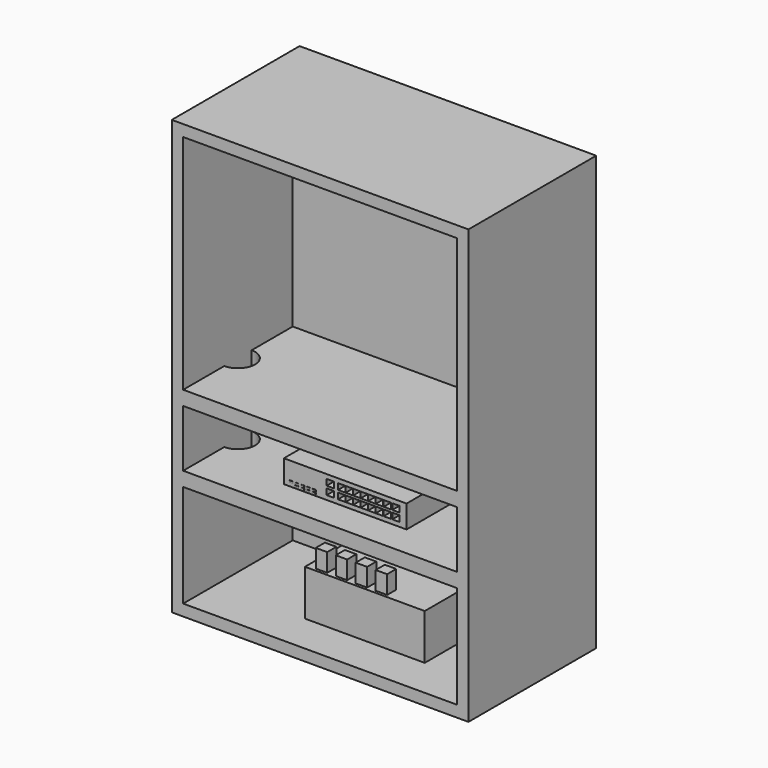
from build123d import *

# Parameters (mm, degrees)
F0_W      = 660.4
F0_H      = 355.6
F1_DEPTH  = 965.2
F2_W      = 609.6
F2_H      = 914.4
F3_DEPTH  = 304.8
F4_W      = 609.6
F4_H      = 31.75
F5_DEPTH  = 304.8
F6_W      = 266.7
F6_H      = 152.4
F7_DEPTH  = 101.6
F8_W      = 25.4
F8_H      = 25.4
F9_DEPTH  = 40.64
F10_W     = 273.05
F10_H     = 215.9
F11_DEPTH = 50.8
F12_W     = 16
F12_H     = 13.3
F13_DEPTH = 19.05
F12_W_2   = 7.62
F12_H_2   = 3.81
F14_DEPTH = 0.635
F16_DEPTH = 190.5


# Not quite as in the source:
# - a feature names something its author has since deleted; it is built from what else it names


with BuildPart() as f1:
    # F0 (on Top) → F1 (new body)
    with BuildSketch(Plane.XY):
        Rectangle(F0_W, F0_H)
    extrude(amount=F1_DEPTH)

    # F2 (on face) → F3 (cut)
    with BuildSketch(Plane.XZ.offset(177.8)):
        with Locations((0, 482.6)):
            Rectangle(F2_W, F2_H)
    extrude(amount=-F3_DEPTH, mode=Mode.SUBTRACT)

    # F4 (on face) → F5 (join)
    with BuildSketch(Plane.XZ.offset(-127)):
        with Locations((0, 269.875)):
            Rectangle(F4_W, F4_H)
        with Locations((0, 428.625)):
            Rectangle(F4_W, F4_H)
    extrude(amount=F5_DEPTH)

    # F6 (on face) → F7 (join)
    with BuildSketch(Plane.XY.offset(25.4)):
        with Locations((29.1608499646, -13.5529870272)):
            Rectangle(F6_W, F6_H)
    extrude(amount=F7_DEPTH)

    # F8 (on face) → F9 (join)
    with BuildSketch(Plane.XY.offset(127)):
        with Locations((-72.4391500354, -70.7029870272)):
            Rectangle(F8_W, F8_H)
        with Locations((-72.4391500354, 43.5970129728)):
            Rectangle(F8_W, F8_H)
        with Locations((-27.9891500354, -70.7029870272)):
            Rectangle(F8_W, F8_H)
        with Locations((-27.9891500354, 43.5970129728)):
            Rectangle(F8_W, F8_H)
        with Locations((16.4608499646, -70.7029870272)):
            Rectangle(F8_W, F8_H)
        with Locations((16.4608499646, 43.5970129728)):
            Rectangle(F8_W, F8_H)
        with Locations((60.9108499646, -70.7029870272)):
            Rectangle(F8_W, F8_H)
        with Locations((60.9108499646, 43.5970129728)):
            Rectangle(F8_W, F8_H)
    extrude(amount=F9_DEPTH)

    # F10 (on face) → F11 (join)
    with BuildSketch(Plane.XY.offset(285.75)):
        Rectangle(F10_W, F10_H)
    extrude(amount=F11_DEPTH)

    # F12 (on face) → F13 (cut)
    with BuildSketch(Plane.XZ.offset(107.95)):
        with Locations((112.775, 301.9346)):
            Rectangle(F12_W, F12_H)
        with Locations((112.775, 320.375)):
            Rectangle(F12_W, F12_H)
        with Locations((93.725, 320.375)):
            Rectangle(F12_W, F12_H)
        with Locations((-33.275, 301.9346)):
            Rectangle(F12_W, F12_H)
        with Locations((93.725, 301.9346)):
            Rectangle(F12_W, F12_H)
        with Locations((-7.875, 320.375)):
            Rectangle(F12_W, F12_H)
        with Locations((-7.875, 301.9346)):
            Rectangle(F12_W, F12_H)
        with Locations((8.889, 320.375)):
            Rectangle(F12_W, F12_H)
        with Locations((8.889, 301.9346)):
            Rectangle(F12_W, F12_H)
        with Locations((25.653, 320.375)):
            Rectangle(F12_W, F12_H)
        with Locations((25.653, 301.9346)):
            Rectangle(F12_W, F12_H)
        with Locations((42.417, 320.375)):
            Rectangle(F12_W, F12_H)
        with Locations((42.417, 301.9346)):
            Rectangle(F12_W, F12_H)
        with Locations((59.181, 320.375)):
            Rectangle(F12_W, F12_H)
        with Locations((59.181, 301.9346)):
            Rectangle(F12_W, F12_H)
        with Locations((75.945, 320.375)):
            Rectangle(F12_W, F12_H)
        with Locations((75.945, 301.9346)):
            Rectangle(F12_W, F12_H)
        with Locations((-33.275, 320.375)):
            Rectangle(F12_W, F12_H)
    extrude(amount=-F13_DEPTH, mode=Mode.SUBTRACT)

    # F12 (on face) → F14 (join, symmetric)
    with BuildSketch(Plane.XZ.offset(107.95)):
        with Locations((-120.015, 295.9252057362)):
            Rectangle(F12_W_2, F12_H_2)
        with Locations((-107.315, 295.9252057362)):
            Rectangle(F12_W_2, F12_H_2)
        with Locations((-94.615, 295.9252057362)):
            Rectangle(F12_W_2, F12_H_2)
        with Locations((-81.915, 295.9252057362)):
            Rectangle(F12_W_2, F12_H_2)
        with Locations((-69.215, 295.9252057362)):
            Rectangle(F12_W_2, F12_H_2)
        with Locations((-81.915, 290.3372057362)):
            Rectangle(F12_W_2, F12_H_2)
        with Locations((-107.315, 290.3372057362)):
            Rectangle(F12_W_2, F12_H_2)
        with Locations((-69.215, 290.3372057362)):
            Rectangle(F12_W_2, F12_H_2)
        with Locations((-94.615, 290.3372057362)):
            Rectangle(F12_W_2, F12_H_2)
    extrude(amount=F14_DEPTH, both=True)

    # F15 (on face) → F16 (cut)
    with BuildSketch(Plane.XY.offset(444.5)):
        with BuildLine():
            ThreePointArc((-304.8, -63.5), (-266.7, -25.4), (-304.8, 12.7))
            Line((-304.8, 12.7), (-304.8, -63.5))
        make_face()
        with BuildLine():
            Line((304.8, -63.5), (304.8, 12.7))
            ThreePointArc((304.8, 12.7), (266.7, -25.4), (304.8, -63.5))
        make_face()
    extrude(amount=-F16_DEPTH, mode=Mode.SUBTRACT)


solid = f1.part
